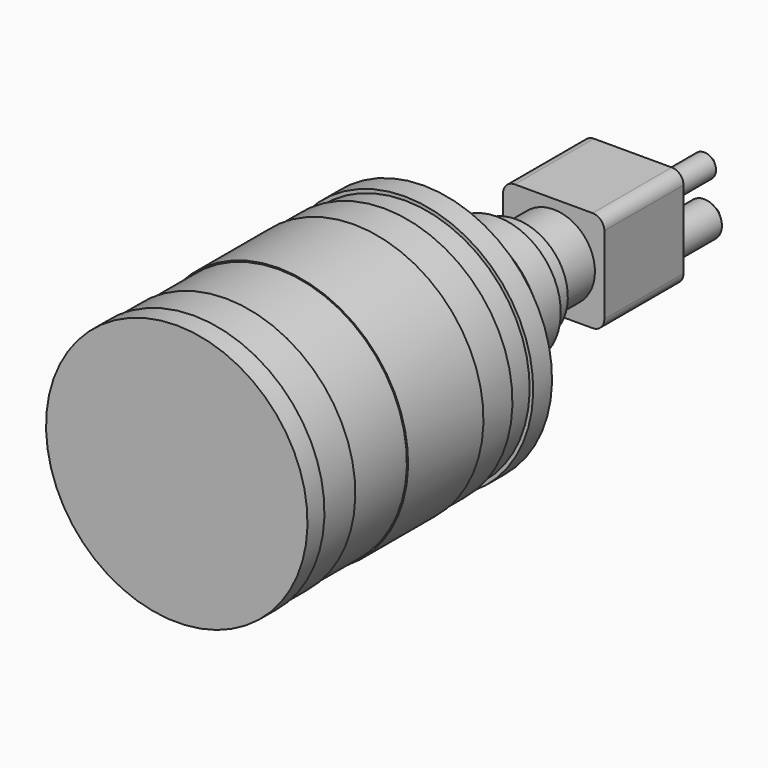
from build123d import *

# Parameters (mm, degrees)
F2_R     = 17.5
F3_DEPTH = 42
F4_R     = 5
F4_R_2   = 7.5
F5_DEPTH = 30
F6_SIZE  = 5


with BuildPart() as f1:
    # F0 (on Right) → F1 (revolve)
    with BuildSketch(Plane.YZ):
        Polygon((-113.8845806535, 55.5), (-113.8845806535, 0), (86.1154193465, 0), (86.1154193465, 17.5), (66.1154193465, 17.5), (66.1154193465, 22), (56.1154193465, 22), (56.1154193465, 27), (41.1154193465, 27), (41.1154193465, 25), (37.1154193465, 25), (37.1154193465, 34), (17.1154193465, 34), (17.1154193465, 54.5), (7.1154193465, 54.5), (7.1154193465, 53), (-3.8845806535, 53), (-3.8845806535, 54.5), (-19.8845806535, 54.5), (-19.8845806535, 55), (-59.8845806535, 55), (-59.8845806535, 54.5), (-87.8845806535, 54.5), (-87.8845806535, 55), (-104.8845806535, 55), (-104.8845806535, 55.5), align=None)
    revolve(axis=Axis((0, -10.2711766958, 0), (0, 1, 0)))


with BuildPart() as f3:
    # F2 (on face) → F3 (new body)
    with BuildSketch(Plane(origin=(0, 86.1154193465, 0), x_dir=(-1, 0, 0), z_dir=(0, 1, 0))):
        with BuildLine():
            Line((16.5, 21.5), (-16.5, 21.5))
            ThreePointArc((-16.5, 21.5), (-20.0355339059, 20.0355339059), (-21.5, 16.5))
            Line((-21.5, 16.5), (-21.5, -16.5))
            ThreePointArc((-21.5, -16.5), (-20.0355339059, -20.0355339059), (-16.5, -21.5))
            Line((-16.5, -21.5), (16.5, -21.5))
            ThreePointArc((16.5, -21.5), (20.0355339059, -20.0355339059), (21.5, -16.5))
            Line((21.5, -16.5), (21.5, 16.5))
            ThreePointArc((21.5, 16.5), (20.0355339059, 20.0355339059), (16.5, 21.5))
        make_face()
        Circle(F2_R, mode=Mode.SUBTRACT)
        Circle(F2_R)
    extrude(amount=F3_DEPTH)

    # F4 (on face) → F5 (join)
    with BuildSketch(Plane(origin=(0, 128.1154193465, 0), x_dir=(-1, 0, 0), z_dir=(0, 1, 0))):
        with Locations((-10.3259523134, 9.9727134464)):
            Circle(F4_R)
        with Locations((-10.3259523134, -10.0272865536)):
            Circle(F4_R_2)
        with Locations((11.3842158583, -10.0272865536)):
            Circle(F4_R_2)
    extrude(amount=F5_DEPTH)

    # F6
    f6_edges = [f3.edges().sort_by_distance(p)[0] for p in [
        (-3.884216, 158.115419, -10.027287),
        (17.825952, 158.115419, -10.027287),
        (15.325952, 158.115419, 9.972713),
    ]]
    chamfer(f6_edges, length=F6_SIZE)


solid = Compound([f1.part, f3.part])
